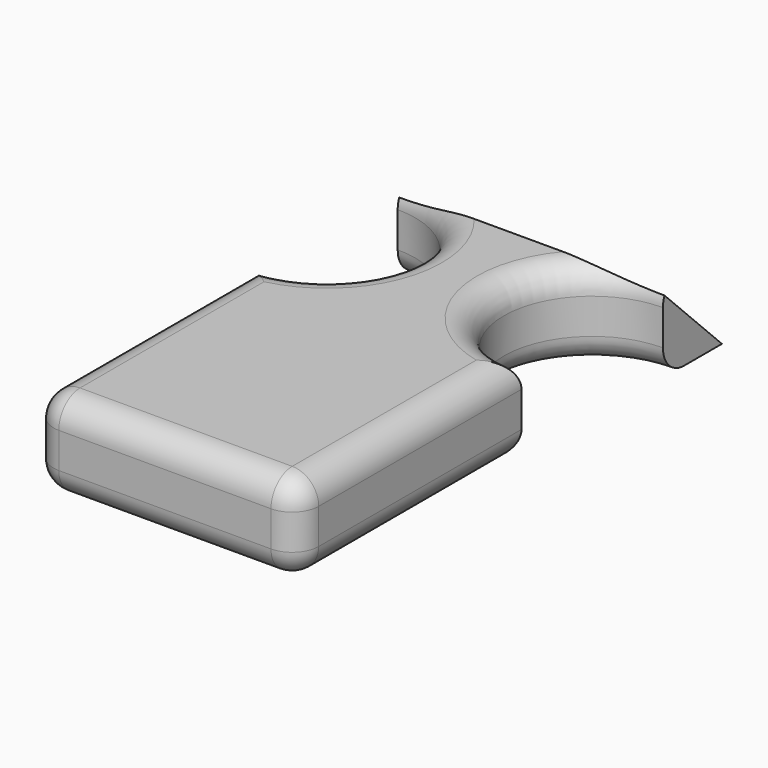
from build123d import *

# Parameters (mm, degrees)
F1_DEPTH    = 10
F2_R        = 3
F3_T1_DEPTH = 81.4336597593


# Not quite as in the source:
# - a fillet or chamfer that OpenCascade refuses, or shapes differently, is made with other operations: its cross-section is extruded or revolved along the edge and cut away or added


with BuildPart() as f1:
    # F0 (on Top) → F1 (new body)
    with BuildSketch(Plane.XY):
        with BuildLine():
            Line((15, 30), (-15, 30))
            Line((-15, 30), (-15, 21.6620222107))
            ThreePointArc((-15, 21.6620222107), (-5, 11.6620222107), (-15, 1.6620222107))
            Line((-15, 1.6620222107), (-15, -30))
            Line((-15, -30), (15, -30))
            Line((15, -30), (15, 1.6620222107))
            ThreePointArc((15, 1.6620222107), (5, 11.6620222107), (15, 21.6620222107))
            Line((15, 21.6620222107), (15, 30))
        make_face()
    extrude(amount=F1_DEPTH)

    # F2
    f2_edges = [f1.edges().sort_by_distance(p)[0] for p in [
        (-5, 11.662022, 10),
        (5, 11.662022, 10),
        (5, 11.662022, 0),
        (-5, 11.662022, 0),
        (0, -30, 0),
        (-15, -14.168989, 0),
        (15, -14.168989, 0),
        (0, -30, 10),
        (15, -14.168989, 10),
        (-15, -14.168989, 10),
        (15, -30, 5),
        (-15, -30, 5),
    ]]
    fillet(f2_edges, radius=F2_R)

    # F3: chamfer of 10 on 1 edges, made by hand

    # F3_s2 → F3_t1 (cut)
    with BuildSketch(Plane.YZ.offset(-40.7168298797)):
        Polygon((20, 10), (30, 0), (30, 10), align=None)
    extrude(amount=F3_T1_DEPTH, mode=Mode.SUBTRACT)


solid = f1.part
